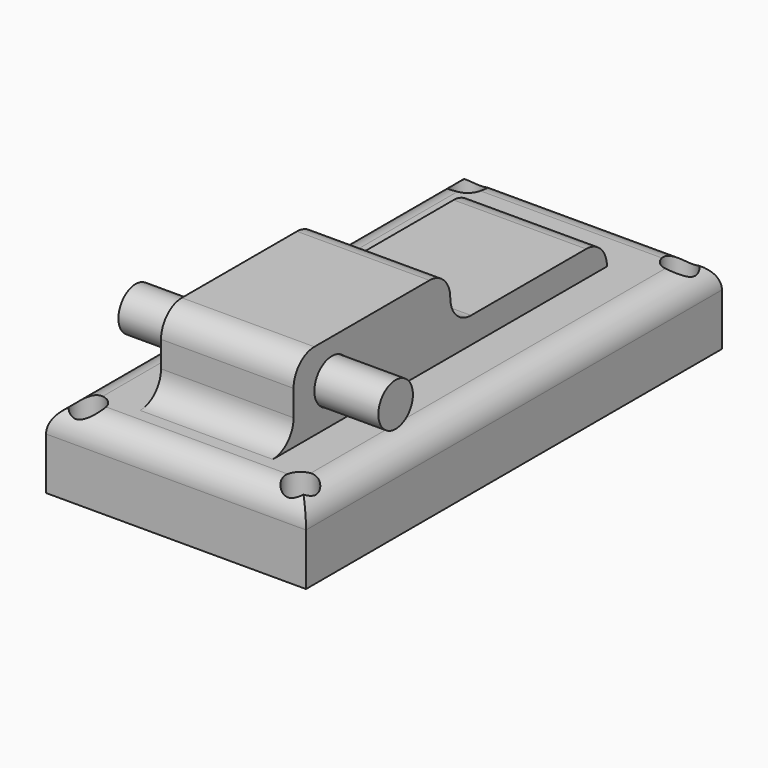
from build123d import *

# Parameters (mm, degrees)
F0_W        = 50
F0_H        = 100
F0_R        = 3
F1_DEPTH    = 15
F0_W_2      = 25.4946034402
F0_H_2      = 37.6753620803
F2_DEPTH    = 20
F3_DEPTH    = 30
F4_T1_DEPTH = 25.4946034402
F4_T3_DEPTH = 50.4946034402
F4_T5_DEPTH = 125
F4_T7_DEPTH = 75
F5_R        = 4.2218085751
F6_DEPTH    = 31.6
F7_R        = 4.1529704456
F8_DEPTH    = 25


# Not quite as in the source:
# - a fillet or chamfer that OpenCascade refuses, or shapes differently, is made with other operations: its cross-section is extruded or revolved along the edge and cut away or added


with BuildPart() as f1:
    # F0 (on Top) → F1 (new body)
    with BuildSketch(Plane.XY):
        Rectangle(F0_W, F0_H)
        with Locations((-20.3956849873, -45.6070154905)):
            Circle(F0_R, mode=Mode.SUBTRACT)
        with Locations((20.3956849873, -45.6070154905)):
            Circle(F0_R, mode=Mode.SUBTRACT)
        with Locations((-20.3956849873, 45.6070154905)):
            Circle(F0_R, mode=Mode.SUBTRACT)
        Polygon((-12.7473017201, 37.6753620803), (12.7473017201, 37.6753620803), (12.7473017201, 0), (12.7473017201, -37.6753620803), (-12.7473017201, -37.6753620803), (-12.7473017201, 0), align=None, mode=Mode.SUBTRACT)
        with Locations((20.3956849873, 45.6070154905)):
            Circle(F0_R, mode=Mode.SUBTRACT)
    extrude(amount=F1_DEPTH)

    # F0 (on Top) → F2 (join)
    with BuildSketch(Plane.XY):
        with Locations((0, 18.8376810402)):
            Rectangle(F0_W_2, F0_H_2)
    extrude(amount=F2_DEPTH)

    # F0 (on Top) → F3 (join)
    with BuildSketch(Plane.XY):
        with Locations((0, -18.8376810402)):
            Rectangle(F0_W_2, F0_H_2)
    extrude(amount=F3_DEPTH)

    # F4: fillet of radius 5 on 9 edges, made by hand

    # F4_s2 → F4_t1 (join)
    with BuildSketch(Plane.YZ.offset(-12.7473017201)):
        with BuildLine():
            ThreePointArc((0, 25), (1.4644660941, 21.4644660941), (5, 20))
            Line((5, 20), (0, 20))
            Line((0, 20), (0, 25))
        make_face()
        with BuildLine():
            ThreePointArc((-42.6753620803, 15), (-39.1398281744, 16.4644660941), (-37.6753620803, 20))
            Line((-37.6753620803, 20), (-37.6753620803, 15))
            Line((-37.6753620803, 15), (-42.6753620803, 15))
        make_face()
    extrude(amount=F4_T1_DEPTH)

    # F4_s4 → F4_t3 (cut)
    with BuildSketch(Plane.YZ.offset(-25.2473017201)):
        with BuildLine():
            ThreePointArc((-5, 30), (-1.4644660941, 28.5355339059), (0, 25))
            Line((0, 25), (0, 30))
            Line((0, 30), (-5, 30))
        make_face()
        with BuildLine():
            ThreePointArc((32.6753620803, 20), (36.2108959863, 18.5355339059), (37.6753620803, 15))
            Line((37.6753620803, 15), (37.6753620803, 20))
            Line((37.6753620803, 20), (32.6753620803, 20))
        make_face()
        with BuildLine():
            ThreePointArc((-37.6753620803, 25), (-36.2108959863, 28.5355339059), (-32.6753620803, 30))
            Line((-32.6753620803, 30), (-37.6753620803, 30))
            Line((-37.6753620803, 30), (-37.6753620803, 25))
        make_face()
    extrude(amount=F4_T3_DEPTH, mode=Mode.SUBTRACT)

    # F4_s6 → F4_t5 (cut)
    with BuildSketch(Plane.XZ.offset(-62.5)):
        with BuildLine():
            ThreePointArc((-20, 15), (-23.5355339059, 13.5355339059), (-25, 10))
            Line((-25, 10), (-25, 15))
            Line((-25, 15), (-20, 15))
        make_face()
        with BuildLine():
            ThreePointArc((25, 10), (23.5355339059, 13.5355339059), (20, 15))
            Line((20, 15), (25, 15))
            Line((25, 15), (25, 10))
        make_face()
    extrude(amount=F4_T5_DEPTH, mode=Mode.SUBTRACT)

    # F4_s8 → F4_t7 (cut)
    with BuildSketch(Plane.YZ.offset(-37.5)):
        with BuildLine():
            ThreePointArc((-45, 15), (-48.5355339059, 13.5355339059), (-50, 10))
            Line((-50, 10), (-50, 15))
            Line((-50, 15), (-45, 15))
        make_face()
        with BuildLine():
            ThreePointArc((45, 15), (48.5355339059, 13.5355339059), (50, 10))
            Line((50, 10), (50, 15))
            Line((50, 15), (45, 15))
        make_face()
    extrude(amount=F4_T7_DEPTH, mode=Mode.SUBTRACT)

    # F5 (on face) → F6 (cut)
    with BuildSketch(Plane.YZ.offset(12.7473017201)):
        with Locations((-28.4535535052, 22.5)):
            Circle(F5_R)
    extrude(amount=-F6_DEPTH, mode=Mode.SUBTRACT)


with BuildPart() as f8:
    # F7 (on Right) → F8 (new body, symmetric)
    with BuildSketch(Plane.YZ):
        with Locations((-28.4535535052, 22.5)):
            Circle(F7_R)
    extrude(amount=F8_DEPTH, both=True)


solid = Compound([f1.part, f8.part])
